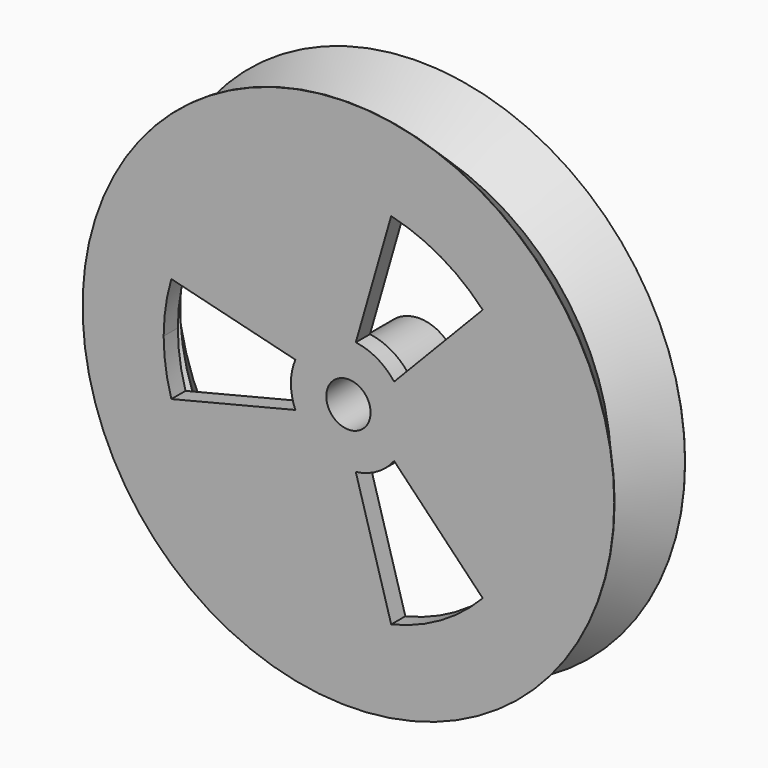
from build123d import *

# Parameters (mm, degrees)
F0_R     = 76.2
F1_DEPTH = 25.4
F4_R     = 6.35
F5_DEPTH = 25.4
F6_T     = 5.08
F8_DEPTH = 5.081


# Not quite as in the source:
# - a shell that OpenCascade refuses in one call is made with other operations: the cavity is built on its own and cut out


with BuildPart() as f1:
    # F0 (on Front) → F1 (new body)
    with BuildSketch(Plane.XZ):
        Circle(F0_R)
    extrude(amount=F1_DEPTH)

    # F2 (on Right) → F3 (revolve, cut)
    with BuildSketch(Plane.YZ):
        Polygon((-12.7, 65.1145875454), (0, 76.22641325), (-12.7, 76.22641325), (-25.3041852266, 76.22641325), align=None)
    revolve(axis=Axis((0, -25.4, 0), (0, -1, 0)), mode=Mode.SUBTRACT)

    # F4 (on face) → F5 (cut)
    with BuildSketch(Plane.XZ.offset(25.4)):
        Circle(F4_R)
    extrude(amount=-F5_DEPTH, mode=Mode.SUBTRACT)

    # F6: shell of thickness 5.08, made by hand


with BuildPart() as f6_core1:
    # F6_t2: copy of F1
    add(f1.part)

    # the walls: a layer under each face that stays
    f6_faces = [f6_core1.faces().sort_by_distance(p)[0] for p in [
        (-76.2, -0.0150942016, 0),
        (0, -6.3650942016, -70.6572937727),
        (-6.35, -12.7, 0),
        (0, -18.9871122894, -70.6572937727),
        (-50.8, -25.4, -50.8),
        (-76.2, -25.3371122894, 0),
    ]]
    thicken(f6_faces, amount=-F6_T, mode=Mode.SUBTRACT)

    # F6_s3 → F6_t4 (revolve, cut)
    with BuildSketch(Plane.YZ):
        Polygon((-12.6998566811, 65.1909254772), (-9.3549115607, 61.2913973417), (-12.712693419, 58.3535164942), (-16.0594203306, 61.3039845692), align=None)
    revolve(axis=Axis((0, -12.7, 0), (0, -1, 0)), mode=Mode.SUBTRACT)


with BuildPart() as f1_1:
    add(f1.part)

    # what is left inside the walls is the cavity
    f6_cavity = [f6_core1.part.solids().sort_by_distance(p)[0] for p in [
        (0, -0.0508, -23.158816),
    ]]
    add(f6_cavity, mode=Mode.SUBTRACT)

    # F7 (on face) → F8 (cut, through all)
    with BuildSketch(Plane(origin=(0, -20.32, 0), x_dir=(-1, 0, 0), z_dir=(0, 1, 0))):
        with BuildLine():
            ThreePointArc((50.750755659, -15.1466698341), (52.4068897458, -7.6536732487), (52.9628247644, 0))
            ThreePointArc((52.9628247644, 0), (52.4068897458, 7.6536732487), (50.750755659, 15.1466698341))
            Line((50.750755659, 15.1466698341), (15.2094055185, 6.3428222009))
            ThreePointArc((15.2094055185, 6.3428222009), (16.1584836664, 3.2343183675), (16.4789990503, 0))
            ThreePointArc((16.4789990503, 0), (16.1584836664, -3.2343183675), (15.2094055185, -6.3428222009))
            Line((15.2094055185, -6.3428222009), (50.750755659, -15.1466698341))
        make_face()
        with BuildLine():
            ThreePointArc((-38.4927786886, -36.3781087449), (-26.4814123822, -45.8671517021), (-12.2579769704, -51.524778579))
            Line((-12.2579769704, -51.524778579), (-2.1116576016, -16.343142656))
            ThreePointArc((-2.1116576016, -16.343142656), (-8.2394995251, -14.2712318065), (-13.0977479169, -10.000320455))
            Line((-13.0977479169, -10.000320455), (-38.4927786886, -36.3781087449))
        make_face()
        with BuildLine():
            Line((-2.1116576016, 16.343142656), (-12.2579769704, 51.524778579))
            ThreePointArc((-12.2579769704, 51.524778579), (-26.4814123822, 45.8671517021), (-38.4927786886, 36.3781087449))
            Line((-38.4927786886, 36.3781087449), (-13.0977479169, 10.000320455))
            ThreePointArc((-13.0977479169, 10.000320455), (-8.2394995251, 14.2712318065), (-2.1116576016, 16.343142656))
        make_face()
    extrude(amount=-F8_DEPTH, mode=Mode.SUBTRACT)


solid = f1_1.part
